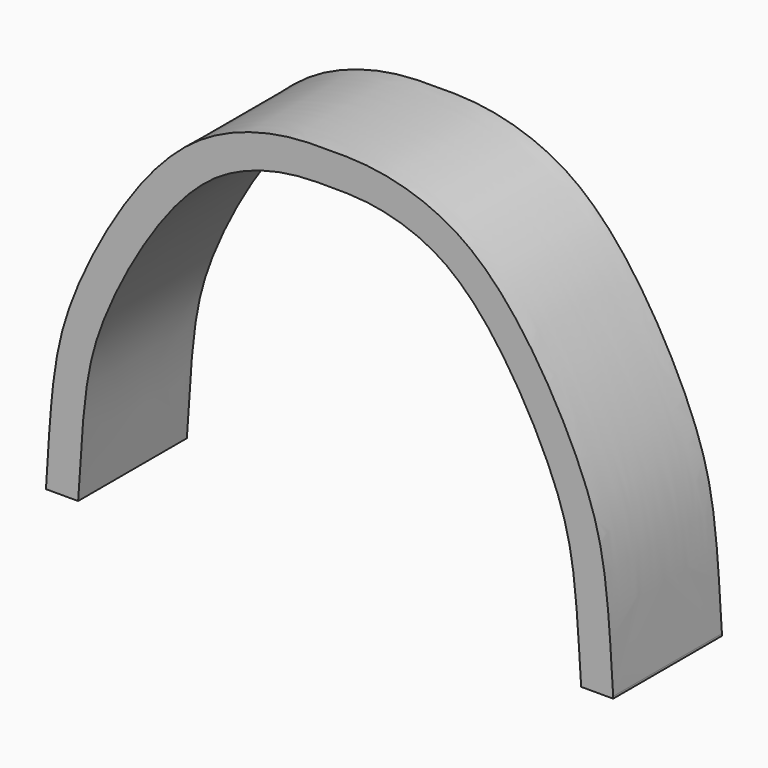
from build123d import *

# Parameters (mm, degrees)
F1_DEPTH = 12.7


# Not quite as in the source:
# - the dataset's text gives a spline's control points without its knots; the knots are read off the source's solid


with BuildPart() as f1:
    # F0 (on Front) → F1 (new body)
    with BuildSketch(Plane.XZ):
        with BuildLine():
            Line((-2.9937300809, 0), (0, 0))
            add(Edge.make_bspline(
                [(0, 0), (0.2247518646, 3.4708543076), (0.5318348568, 9.7099533004), (2.1678993745, 15.7836377097), (6.3257813429, 24.0181350284), (12.23456879, 31.3258977025), (19.0045682902, 33.4480303309), (21.8033740862, 33.5), (23.5, 33.5)],
                knots=[0, 0, 0, 0, 0.1904027648, 0.3424874988, 0.5268393176, 0.7141316637, 0.8703898231, 1, 1, 1, 1], degree=3))
            add(Edge.make_bspline(
                [(47, 0), (46.7752481354, 3.4708543076), (46.4681651432, 9.7099533004), (44.8321006255, 15.7836377097), (40.6742186571, 24.0181350284), (34.76543121, 31.3258977025), (27.9954317098, 33.4480303309), (25.1966259138, 33.5), (23.5, 33.5)],
                knots=[0, 0, 0, 0, 0.1904027648, 0.3424874988, 0.5268393176, 0.7141316637, 0.8703898231, 1, 1, 1, 1], degree=3))
            Line((47, 0), (49.9937300809, 0))
            Line((49.9937300809, 0), (49.9937300809, 0.1938561397))
            add(Edge.make_bspline(
                [(49.9937300809, 0.1938561397), (49.9206107807, 1.3230411561), (49.7847205721, 3.6012238657), (49.5505077824, 6.9307082666), (49.2741056202, 9.5303506796), (48.9610556104, 11.451889245), (48.669643101, 12.8298378292), (48.3125227684, 14.1731591899), (47.8842532657, 15.5039883991), (47.3827375221, 16.8463006194), (46.8005209225, 18.2415097274), (46.1391833251, 19.6847282983), (45.1588220426, 21.652476332), (44.0380137387, 23.6586982796), (42.7954602194, 25.6392623644), (41.4671196396, 27.5937880735), (39.9958864522, 29.4759685035), (38.3534032951, 31.2009700755), (37.2449881143, 32.1948140337), (36.3043625762, 32.9248008221), (35.5658502311, 33.4379606917), (34.8158339023, 33.899739938), (33.8104650793, 34.449811273), (32.5531054649, 35.0221257848), (31.0753374909, 35.5477180543), (29.8935182494, 35.869862714), (28.9901351243, 36.0683555772), (28.1214790819, 36.2303075607), (27.0833725979, 36.3726079701), (25.8874908606, 36.4630755765), (24.715206538, 36.4973264093), (23.9157663812, 36.5), (23.5, 36.5)],
                knots=[0, 0, 0, 0, 0.0625, 0.125, 0.1875, 0.21875, 0.25, 0.28125, 0.3125, 0.34375, 0.375, 0.40625, 0.4375, 0.5, 0.53125, 0.5625, 0.625, 0.65625, 0.6875, 0.703125, 0.71875, 0.734375, 0.75, 0.78125, 0.8125, 0.84375, 0.859375, 0.875, 0.90625, 0.9375, 0.96875, 1, 1, 1, 1], degree=3))
            add(Edge.make_bspline(
                [(-2.9937300809, 0.1938561397), (-2.9206107807, 1.3230411561), (-2.7847205721, 3.6012238657), (-2.5505077824, 6.9307082666), (-2.2741056202, 9.5303506796), (-1.9610556104, 11.451889245), (-1.669643101, 12.8298378292), (-1.3125227684, 14.1731591899), (-0.8842532657, 15.5039883991), (-0.3827375221, 16.8463006194), (0.1994790775, 18.2415097274), (0.8608166749, 19.6847282983), (1.8411779574, 21.652476332), (2.9619862613, 23.6586982796), (4.2045397806, 25.6392623644), (5.5328803604, 27.5937880735), (7.0041135478, 29.4759685035), (8.6465967049, 31.2009700755), (9.7550118857, 32.1948140337), (10.6956374238, 32.9248008221), (11.4341497689, 33.4379606917), (12.1841660977, 33.899739938), (13.1895349207, 34.449811273), (14.4468945351, 35.0221257848), (15.9246625091, 35.5477180543), (17.1064817506, 35.869862714), (18.0098648757, 36.0683555772), (18.8785209181, 36.2303075607), (19.9166274021, 36.3726079701), (21.1125091394, 36.4630755765), (22.284793462, 36.4973264093), (23.0842336188, 36.5), (23.5, 36.5)],
                knots=[0, 0, 0, 0, 0.0625, 0.125, 0.1875, 0.21875, 0.25, 0.28125, 0.3125, 0.34375, 0.375, 0.40625, 0.4375, 0.5, 0.53125, 0.5625, 0.625, 0.65625, 0.6875, 0.703125, 0.71875, 0.734375, 0.75, 0.78125, 0.8125, 0.84375, 0.859375, 0.875, 0.90625, 0.9375, 0.96875, 1, 1, 1, 1], degree=3))
            Line((-2.9937300809, 0.1938561397), (-2.9937300809, 0))
        make_face()
    extrude(amount=F1_DEPTH)


solid = f1.part
